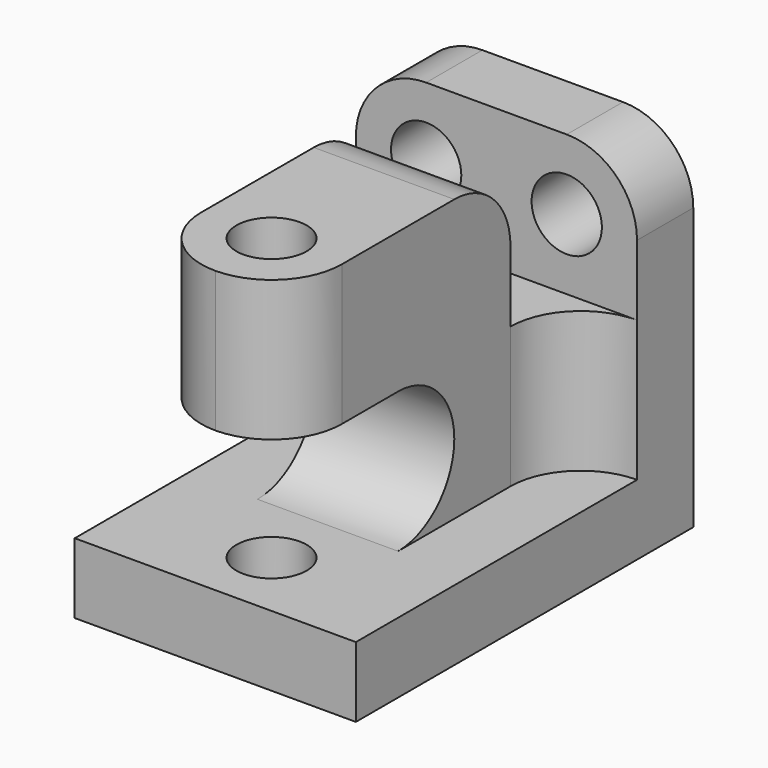
from build123d import *

# Parameters (mm, degrees)
F1_DEPTH  = 20
F3_DEPTH  = 10
F5_DEPTH  = 20
F6_R      = 10
F6_R_2    = 9.99999
F8_D      = 10
F10_D     = 10
F10_DEPTH = 10.001


# Not quite as in the source:
# - a fillet or chamfer is up to 0.001 mm smaller than in the source, because OpenCascade refuses the exact size


with BuildPart() as f1:
    # F0 (on Right) → F1 (new body, symmetric)
    with BuildSketch(Plane.YZ):
        Polygon((-60, 0), (0, 0), (0, 50), (-10, 50), (-10, 10), (-60, 10), align=None)
    extrude(amount=F1_DEPTH, both=True)

    # F2 (on Right) → F3 (join, symmetric)
    with BuildSketch(Plane.YZ):
        with BuildLine():
            Line((-60, 10), (-10, 10))
            Line((-10, 10), (-10, 30))
            Line((-10, 30), (-20, 30))
            Line((-20, 30), (-20, 40))
            ThreePointArc((-20, 40), (-22.9289321881, 47.0710678119), (-30, 50))
            Line((-30, 50), (-60, 50))
            Line((-60, 50), (-60, 10))
        make_face()
    extrude(amount=F3_DEPTH, both=True)

    # F4 (on face) → F5 (cut, through all)
    with BuildSketch(Plane.YZ.offset(10)):
        with BuildLine():
            Line((-60, 30), (-60, 10))
            Line((-60, 10), (-40, 10))
            ThreePointArc((-40, 10), (-30, 20), (-40, 30))
            Line((-40, 30), (-60, 30))
        make_face()
    extrude(amount=-F5_DEPTH, mode=Mode.SUBTRACT)

    # F6 (call 1 of 6: OpenCascade refuses the feature's edges together)
    f6_edges = [f1.edges().sort_by_distance(p)[0] for p in [
        (-20, -5, 50),
    ]]
    fillet(f6_edges, radius=F6_R)

    # F6#2 (call 2 of 6)
    f6_2_edges = [f1.edges().sort_by_distance(p)[0] for p in [
        (20, -5, 50),
    ]]
    fillet(f6_2_edges, radius=F6_R)

    # F6#3 (call 3 of 6)
    f6_3_edges = [f1.edges().sort_by_distance(p)[0] for p in [
        (-10, -60, 40),
    ]]
    fillet(f6_3_edges, radius=F6_R)

    # F6#4 (call 4 of 6) (radius 10 in the source; OpenCascade refuses exactly that, so slightly less here)
    f6_4_edges = [f1.edges().sort_by_distance(p)[0] for p in [
        (10, -60, 40),
    ]]
    fillet(f6_4_edges, radius=F6_R_2)

    # F6#5 (call 5 of 6) (radius 10 in the source; OpenCascade refuses exactly that, so slightly less here)
    f6_5_edges = [f1.edges().sort_by_distance(p)[0] for p in [
        (10, -10, 20),
    ]]
    fillet(f6_5_edges, radius=F6_R_2)

    # F6#6 (call 6 of 6) (radius 10 in the source; OpenCascade refuses exactly that, so slightly less here)
    f6_6_edges = [f1.edges().sort_by_distance(p)[0] for p in [
        (-10, -10, 20),
    ]]
    fillet(f6_6_edges, radius=F6_R_2)

    # F8 (through all)
    with Locations(Plane.XY.offset(50)):
        with Locations((0, -50)):
            Hole(F8_D / 2)

    # F10 (through all, one way)
    with BuildSketch(Plane.XZ.offset(10)):
        with Locations((-10, 40), (10, 40)):
            Circle(F10_D / 2)
    extrude(amount=-F10_DEPTH, mode=Mode.SUBTRACT)


solid = f1.part
